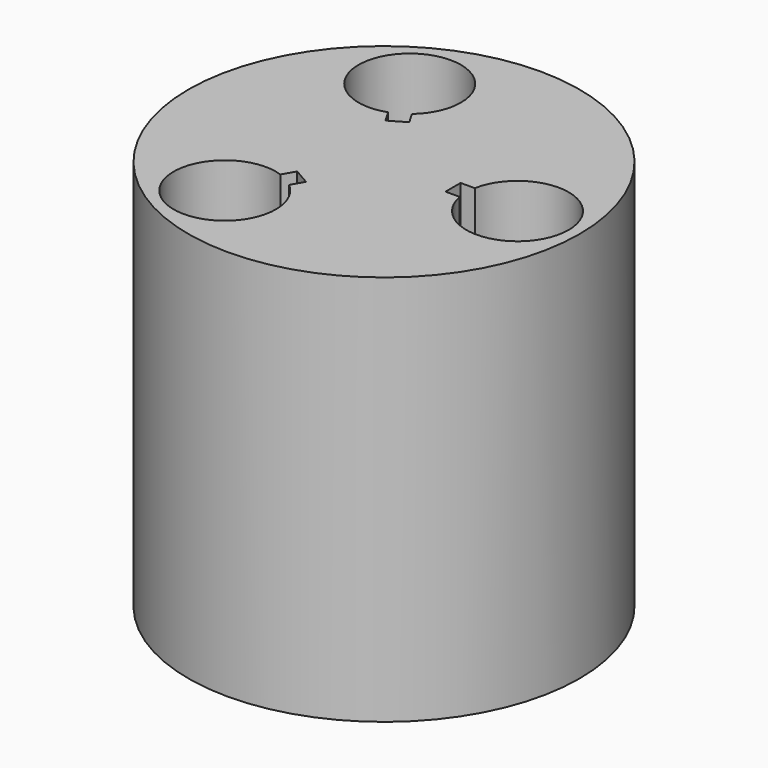
from build123d import *

# Parameters (mm, degrees)
F0_R            = 42.5
F1_DEPTH        = 85
F3_DEPTH        = 85.001
F3_COPIES_COUNT = 3


# Not quite as in the source:
# - a pattern or mirror of a feature is missing from the dataset's text; its kind, count and spacing are read off the source's solid


with BuildPart() as f1:
    # F0 (on Top) → F1 (new body)
    with BuildSketch(Plane.XY):
        Circle(F0_R)
    extrude(amount=F1_DEPTH)

    # F2 (on face) → F3 (cut, through all)
    with BuildSketch(Plane.XY.offset(85)):
        with BuildLine():
            Line((15, -2.05), (18.0782255906, -2.05))
            ThreePointArc((18.0782255906, -2.05), (40.1125, 0), (18.0782255906, 2.05))
            Line((18.0782255906, 2.05), (15, 2.05))
            Line((15, 2.05), (15, -2.05))
        make_face()
    f3 = extrude(amount=-F3_DEPTH, mode=Mode.SUBTRACT)

    # F3_copies: F3 ×3 about axis
    f3_copies_axis = Axis((0, 0, 0), (0, 0, 1))
    for i in range(1, F3_COPIES_COUNT):
        add(f3.rotate(f3_copies_axis, i * 360 / F3_COPIES_COUNT), mode=Mode.SUBTRACT)


solid = f1.part
